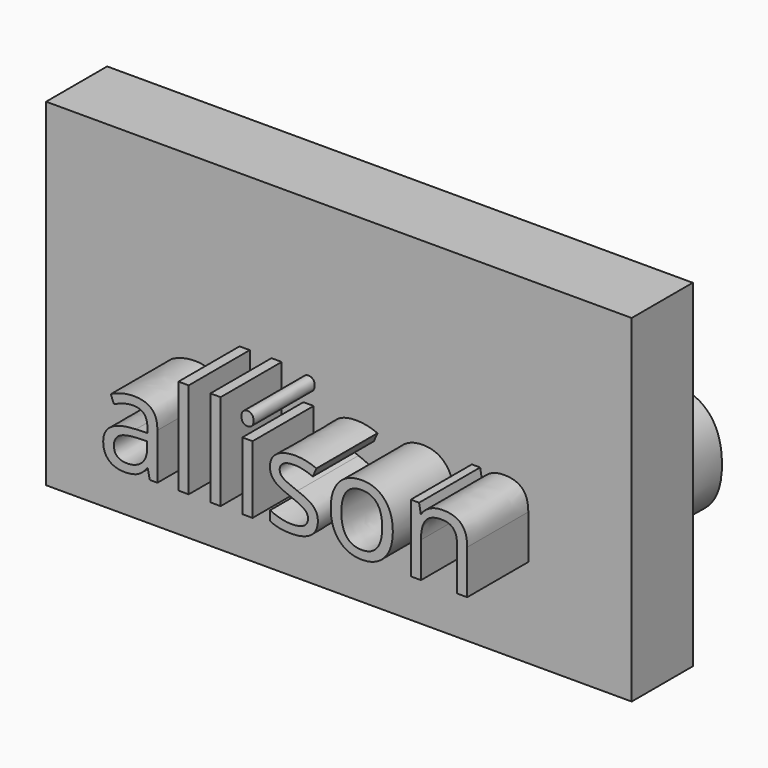
from build123d import *

# Parameters (mm, degrees)
F0_W         = 194.8468089104
F0_H         = 112.3622730374
F1_DEPTH     = 25.4
F2_TEXT_SIZE = 42.0060131647
F3_DEPTH     = 25.4
F4_TEXT_SIZE = 65.0794115952
F5_DEPTH     = 25.4


# Not quite as in the source:
# - Text() gives the source's letters only with a copy of the font that has no kerning and outlines rounded to 1/6400 em; it was checked with that copy


with BuildPart() as f1:
    # F0 (on Front) → F1 (new body)
    with BuildSketch(Plane.XZ):
        with Locations((-5.2009448409, 9.5315463841)):
            Rectangle(F0_W, F0_H)
    extrude(amount=F1_DEPTH)

    # F2 (on face) → F3 (join)
    with BuildSketch(Plane.XZ.offset(25.4)):
        with Locations((-65.2240216732, -16.9433620758)):
            Text('allison', F2_TEXT_SIZE, font='Open Sans', text_align=(TextAlign.LEFT, TextAlign.BOTTOM))
    extrude(amount=F3_DEPTH)

    # F4 (on face) → F5 (join)
    with BuildSketch(Plane(origin=(0, 0, 0), x_dir=(-1, 0, 0), z_dir=(0, 1, 0))):
        with Locations((-85.2730423212, -18.4799749404)):
            Text('cassie', F4_TEXT_SIZE, font='Open Sans', text_align=(TextAlign.LEFT, TextAlign.BOTTOM))
    extrude(amount=F5_DEPTH)


solid = f1.part
